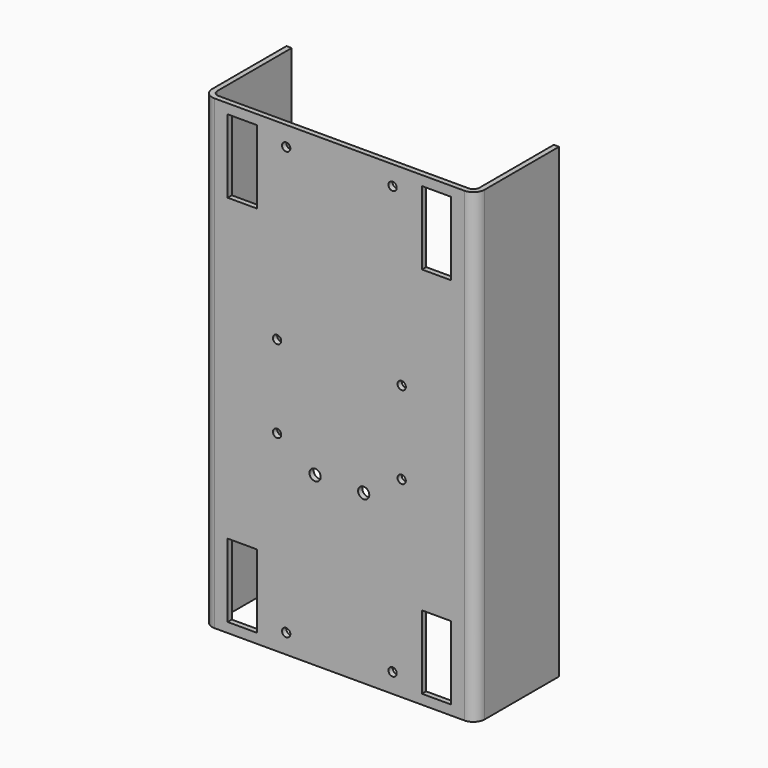
from build123d import *

# Parameters (mm, degrees)
F1_DEPTH = 152.4
F2_R     = 1.98374
F3_R     = 3.69316
F4_W     = 9.5329248
F4_H     = 24
F4_R     = 1.35255
F5_DEPTH = 1.70942
F6_R     = 1.35255
F6_R_2   = 1.8288
F7_DEPTH = 1.70942


with BuildPart() as f1:
    # F0 (on Top) → F1 (new body)
    with BuildSketch(Plane.XY):
        Polygon((0, 32.3337428), (0, 0), (-85.6425008, 0), (-85.6425008, 32.3337428), (-87.3519208, 32.3337428), (-87.3519208, -1.70942), (1.70942, -1.70942), (1.70942, 32.3337428), align=None)
    extrude(amount=F1_DEPTH)

    # F2
    f2_edges = [f1.edges().sort_by_distance(p)[0] for p in [
        (0, 0, 76.2),
        (-85.642501, 0, 76.2),
    ]]
    fillet(f2_edges, radius=F2_R)

    # F3
    f3_edges = [f1.edges().sort_by_distance(p)[0] for p in [
        (1.70942, -1.70942, 76.2),
        (-87.351921, -1.70942, 76.2),
    ]]
    fillet(f3_edges, radius=F3_R)

    # F4 (on face) → F5 (cut, through all)
    with BuildSketch(Plane(origin=(0, 0, 0), x_dir=(-1, 0, 0), z_dir=(0, 1, 0))):
        with Locations((74.5712504, 15.175)):
            Rectangle(F4_W, F4_H)
        with Locations((11.0712504, 15.175)):
            Rectangle(F4_W, F4_H)
        with Locations((11.0712504, 137.225)):
            Rectangle(F4_W, F4_H)
        with Locations((74.5712504, 137.225)):
            Rectangle(F4_W, F4_H)
        with Locations((60.20308, 6.35)):
            Circle(F4_R)
        with Locations((25.4394208, 6.35)):
            Circle(F4_R)
        with Locations((25.4394208, 146.05)):
            Circle(F4_R)
        with Locations((60.20308, 146.05)):
            Circle(F4_R)
    extrude(amount=-F5_DEPTH, mode=Mode.SUBTRACT)

    # F6 (on face) → F7 (cut, through all)
    with BuildSketch(Plane.XZ.offset(1.70942)):
        with Locations((-63.1831604, 89.69375)):
            Circle(F6_R)
        with Locations((-22.4593404, 89.69375)):
            Circle(F6_R)
        with Locations((-22.4593404, 62.70625)):
            Circle(F6_R)
        with Locations((-63.1831604, 62.70625)):
            Circle(F6_R)
        with Locations((-50.7587504, 54.76875)):
            Circle(F6_R_2)
        with Locations((-34.8837504, 54.76875)):
            Circle(F6_R_2)
    extrude(amount=-F7_DEPTH, mode=Mode.SUBTRACT)


solid = f1.part
